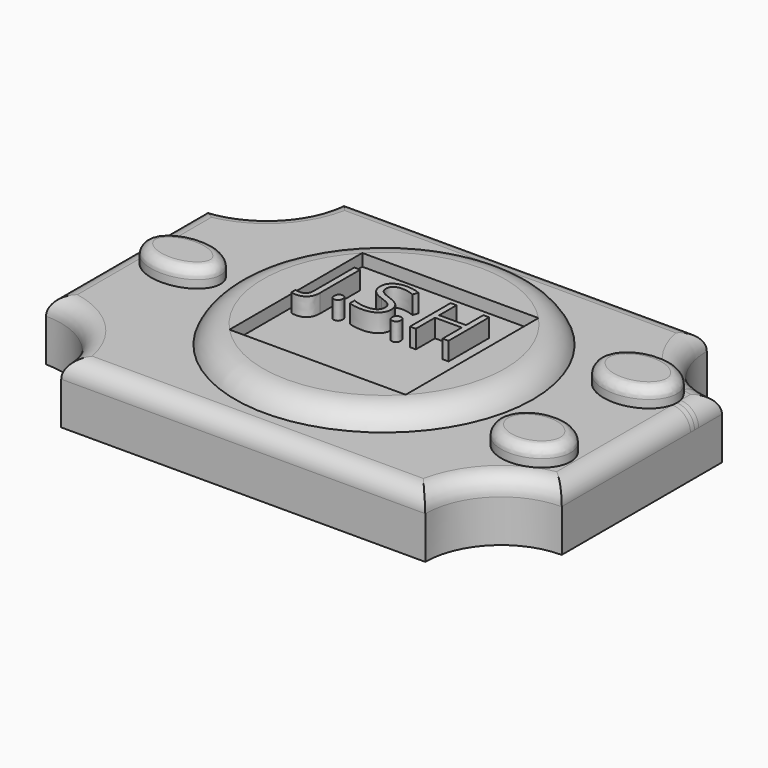
from build123d import *

# Parameters (mm, degrees)
F1_DEPTH      = 10
F2_R          = 24.5371266065
F3_DEPTH      = 3
F4_DEPTH      = 3
F6_W          = 29.0455966875
F6_H          = 27.3695034919
F7_DEPTH      = 2
F9_DEPTH      = 3
F10_R         = 1.6899494937
F12_TEXT_SIZE = 11.7302052786
F13_DEPTH     = 3
F14_R         = 3


# Not quite as in the source:
# - a fillet or chamfer that OpenCascade refuses, or shapes differently, is made with other operations: its cross-section is extruded or revolved along the edge and cut away or added
# - a feature of the source that left no trace in its solid (it failed there, or was rolled back) is left out
# - Text() gives the source's letters only with a copy of the font that has no kerning and outlines rounded to 1/6400 em; it was checked with that copy


with BuildPart() as f1:
    # F0 (on Top) → F1 (new body)
    with BuildSketch(Plane.XY):
        with BuildLine():
            Line((30, 29), (-30, 29))
            ThreePointArc((-30, 29), (-33.6611652352, 20.1611652352), (-42.5, 16.5))
            Line((-42.5, 16.5), (-42.5, -16.5))
            ThreePointArc((-42.5, -16.5), (-33.6611652352, -20.1611652352), (-30, -29))
            Line((-30, -29), (30, -29))
            ThreePointArc((30, -29), (33.6611652352, -20.1611652352), (42.5, -16.5))
            Line((42.5, -16.5), (42.5, 16.5))
            ThreePointArc((42.5, 16.5), (33.6611652352, 20.1611652352), (30, 29))
        make_face()
    extrude(amount=F1_DEPTH)

    # F2 (on face) → F3 (join)
    with BuildSketch(Plane.XY.offset(10)):
        Circle(F2_R)
        with BuildLine():
            ThreePointArc((13.8148347084, 13.8148347084), (18.0499513958, 7.4765346683), (19.5371266065, 0))
            ThreePointArc((19.5371266065, 0), (18.0499513958, -7.4765346683), (13.8148347084, -13.8148347084))
            ThreePointArc((13.8148347084, -13.8148347084), (0, -19.5371266065), (-13.8148347084, -13.8148347084))
            ThreePointArc((-13.8148347084, -13.8148347084), (-19.5371266065, 0), (-13.8148347084, 13.8148347084))
            ThreePointArc((-13.8148347084, 13.8148347084), (0, 19.5371266065), (13.8148347084, 13.8148347084))
        make_face(mode=Mode.SUBTRACT)
    extrude(amount=F3_DEPTH)

    # F4 (add): a face of the model
    f4_faces = [f1.faces().sort_by_distance(p)[0] for p in [
        (0, 0, 10),
    ]]
    extrude(f4_faces, amount=F4_DEPTH)

    # F5: fillet of radius 5 on 1 edges, made by hand

    # F5_s1 → F5_t2 (revolve, cut)
    with BuildSketch(Plane.XZ):
        with BuildLine():
            ThreePointArc((24.5371266065, 10), (22.6931636991, 12.1833001327), (19.9545509116, 13))
            Line((19.9545509116, 13), (24.5371266065, 13))
            Line((24.5371266065, 13), (24.5371266065, 10))
        make_face()
    revolve(axis=Axis((0, 0, 13), (0, 0, 1)), mode=Mode.SUBTRACT)

    # F6 (on face) → F7 (cut)
    with BuildSketch(Plane.XY.offset(13)):
        Rectangle(F6_W, F6_H)
    extrude(amount=-F7_DEPTH, mode=Mode.SUBTRACT)

    # F8 (on face) → F9 (join)
    with BuildSketch(Plane.XY.offset(10)):
        with BuildLine():
            add(Edge.make_bspline(
                [(-26.949954883, 0), (-26.949954883, 7.5344221766), (-36.2713887762, 3.7672110883), (-45.5928226694, 0), (-36.2713887762, -3.7672110883), (-26.949954883, -7.5344221766), (-26.949954883, 0)],
                knots=[0, 0, 0, 2.0943951024, 2.0943951024, 4.1887902048, 4.1887902048, 6.2831853072, 6.2831853072, 6.2831853072], degree=2, weights=[1, 0.5, 1, 0.5, 1, 0.5, 1]))
        make_face()
        with BuildLine():
            add(Edge.make_bspline(
                [(39.5928132931, 10.8537515625), (39.5928132931, 19.5140056004), (29.9499539832, 15.1838785815), (20.3070946733, 10.8537515625), (29.9499539832, 6.5236245436), (39.5928132931, 2.1934975247), (39.5928132931, 10.8537515625)],
                knots=[0, 0, 0, 2.0943951024, 2.0943951024, 4.1887902048, 4.1887902048, 6.2831853072, 6.2831853072, 6.2831853072], degree=2, weights=[1, 0.5, 1, 0.5, 1, 0.5, 1]))
        make_face()
        with BuildLine():
            add(Edge.make_bspline(
                [(39.1642394515, -10.5000028561), (39.1642394515, -1.8397488183), (30.1642409041, -6.1698758372), (21.1642423566, -10.5000028561), (30.1642409041, -14.8301298751), (39.1642394515, -19.160256894), (39.1642394515, -10.5000028561)],
                knots=[0, 0, 0, 2.0943951024, 2.0943951024, 4.1887902048, 4.1887902048, 6.2831853072, 6.2831853072, 6.2831853072], degree=2, weights=[1, 0.5, 1, 0.5, 1, 0.5, 1]))
        make_face()
    extrude(amount=F9_DEPTH)

    # F10
    f10_edges = [f1.edges().sort_by_distance(p)[0] for p in [
        (-39.378533, 0, 13),
        (27.164241, -10.500003, 13),
        (26.735668, 10.853752, 13),
    ]]
    fillet(f10_edges, radius=F10_R)

    # F12 (on face) → F13 (join)
    with BuildSketch(Plane.XY.offset(11)):
        with Locations((-12.681970811, 0)):
            Text('J.S.H', F12_TEXT_SIZE, font='Open Sans', text_align=(TextAlign.LEFT, TextAlign.BOTTOM))
    extrude(amount=F13_DEPTH)

    # F14
    f14_edges = [f1.edges().sort_by_distance(p)[0] for p in [
        (0, 29, 10),
        (-33.661165, 20.161165, 10),
        (-42.5, 0, 10),
        (-33.661165, -20.161165, 10),
        (0, -29, 10),
        (33.661165, -20.161165, 10),
        (42.5, 0, 10),
        (33.661165, 20.161165, 10),
    ]]
    fillet(f14_edges, radius=F14_R)


solid = f1.part
